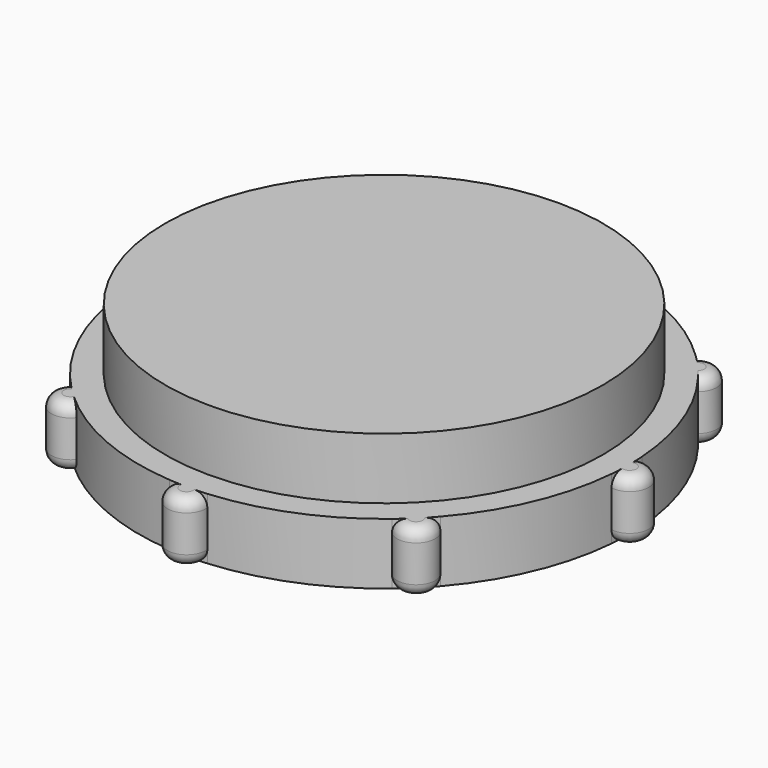
from build123d import *

# Parameters (mm, degrees)
F0_R         = 20
F1_DEPTH     = 5
F2_R         = 17.85
F3_DEPTH     = 5
F4_R         = 1.5514716271
F5_DEPTH     = 5
F6_T4_ANGLE  = 359.64
F6_S5_R      = 20
F6_T6_DEPTH  = 4
F6_T10_ANGLE = 359.64
F6_S11_R     = 20
F6_T12_DEPTH = 4
F6_T16_ANGLE = 359.64
F6_S17_R     = 20
F6_T18_DEPTH = 4
F6_T22_ANGLE = 359.64
F6_S23_R     = 20
F6_T24_DEPTH = 4
F6_T28_ANGLE = 359.64
F6_S29_R     = 20
F6_T30_DEPTH = 4
F6_T34_ANGLE = 359.64
F6_S35_R     = 20
F6_T36_DEPTH = 4
F6_T40_ANGLE = 359.64
F6_S41_R     = 20
F6_T42_DEPTH = 4
F6_T46_ANGLE = 359.64
F6_S47_R     = 20
F6_T48_DEPTH = 4
F6_T52_ANGLE = 359.64
F6_S53_R     = 20
F6_T54_DEPTH = 4
F6_T58_ANGLE = 359.64
F6_S59_R     = 20
F6_T60_DEPTH = 4
F6_T64_ANGLE = 359.64
F6_S65_R     = 20
F6_T66_DEPTH = 4
F6_T70_ANGLE = 359.64
F6_S71_R     = 20
F6_T72_DEPTH = 4
F6_T76_ANGLE = 359.64
F6_S77_R     = 20
F6_T78_DEPTH = 4
F6_T82_ANGLE = 359.64
F6_S83_R     = 20
F6_T84_DEPTH = 4
F6_T88_ANGLE = 359.64
F6_S89_R     = 20
F6_T90_DEPTH = 4
F6_T94_ANGLE = 359.64
F6_S95_R     = 20
F6_T96_DEPTH = 4


# Not quite as in the source:
# - a fillet or chamfer that OpenCascade refuses, or shapes differently, is made with other operations: its cross-section is extruded or revolved along the edge and cut away or added


with BuildPart() as f1:
    # F0 (on Top) → F1 (new body)
    with BuildSketch(Plane.XY):
        Circle(F0_R)
    extrude(amount=F1_DEPTH)

    # F2 (on face) → F3 (join)
    with BuildSketch(Plane.XY.offset(5)):
        Circle(F2_R)
    extrude(amount=F3_DEPTH)

    # F4 (on face) + F2 (on face) → F5 (join)
    with BuildSketch(Plane.XY):
        with Locations((0, -20.1228894293)):
            Circle(F4_R)
        with Locations((13.9962770045, -14.2214773223)):
            Circle(F4_R)
        with Locations((20.1879236847, -0.1935280598)):
            Circle(F4_R)
        with Locations((14.9637199938, 13.2539533079)):
            Circle(F4_R)
        with Locations((0.0650717993, 19.9293233454)):
            Circle(F4_R)
        with Locations((-13.8661321253, 14.6083775908)):
            Circle(F4_R)
        with Locations((-20.2512666583, -0.1935280598)):
            Circle(F4_R)
        with Locations((-13.962876983, -14.5117100328)):
            Circle(F4_R)
    with BuildSketch(Plane.XY.offset(5)):
        Circle(F2_R)
    extrude(amount=F5_DEPTH)

    # F6: fillet of radius 1 on 16 edges, made by hand


with BuildPart() as f6_tool2:
    # F6_s3 → F6_t4 (revolve)
    with BuildSketch(Plane(origin=(-0.0457273893, 0.0437221588, 0), x_dir=(0, 0, 1), z_dir=(0.7227767201, -0.6910816253, 0))):
        with BuildLine():
            ThreePointArc((0, 19.5867422733), (0.2928932188, 18.8796354921), (1, 18.5867422733))
            Line((1, 18.5867422733), (0, 18.5867422733))
            Line((0, 18.5867422733), (0, 19.5867422733))
        make_face()
    revolve(axis=Axis((-13.962876983, -14.5117100328, 0), (0, 0, 1)), revolution_arc=F6_T4_ANGLE)

    # F6_s5 → F6_t6 (cut, symmetric)
    with BuildSketch(Plane.XY.offset(0.5)):
        Circle(F6_S5_R)
    extrude(amount=F6_T6_DEPTH, both=True, mode=Mode.SUBTRACT)


with BuildPart() as f1_1:
    add(f1.part)

    # F6_t1: cut F6_tool2
    add(f6_tool2.part, mode=Mode.SUBTRACT)


with BuildPart() as f6_tool8:
    # F6_s9 → F6_t10 (revolve)
    with BuildSketch(Plane(origin=(0.0632175056, -0.0001986043, 0), x_dir=(0, 0, 1), z_dir=(-0.9999950652, 0.0031415875, 0))):
        with BuildLine():
            ThreePointArc((0, -19.5713184999), (0.2928932188, -18.8642117187), (1, -18.5713184999))
            Line((1, -18.5713184999), (0, -18.5713184999))
            Line((0, -18.5713184999), (0, -19.5713184999))
        make_face()
    revolve(axis=Axis((0, -20.1228894293, 0), (0, 0, -1)), revolution_arc=F6_T10_ANGLE)

    # F6_s11 → F6_t12 (cut, symmetric)
    with BuildSketch(Plane.XY.offset(0.5)):
        Circle(F6_S11_R)
    extrude(amount=F6_T12_DEPTH, both=True, mode=Mode.SUBTRACT)


with BuildPart() as f1_2:
    add(f1_1.part)

    # F6_t7: cut F6_tool8
    add(f6_tool8.part, mode=Mode.SUBTRACT)


with BuildPart() as f6_tool14:
    # F6_s15 → F6_t16 (revolve)
    with BuildSketch(Plane(origin=(0.044815932, 0.0438299518, 0), x_dir=(0, 0, 1), z_dir=(-0.7149274846, -0.6991986068, 0))):
        with BuildLine():
            ThreePointArc((0, -19.4020307643), (0.2928932188, -18.6949239831), (1, -18.4020307643))
            Line((1, -18.4020307643), (0, -18.4020307643))
            Line((0, -18.4020307643), (0, -19.4020307643))
        make_face()
    revolve(axis=Axis((13.9962770045, -14.2214773223, 0), (0, 0, -1)), revolution_arc=F6_T16_ANGLE)

    # F6_s17 → F6_t18 (cut, symmetric)
    with BuildSketch(Plane.XY.offset(0.5)):
        Circle(F6_S17_R)
    extrude(amount=F6_T18_DEPTH, both=True, mode=Mode.SUBTRACT)


with BuildPart() as f1_3:
    add(f1_2.part)

    # F6_t13: cut F6_tool14
    add(f6_tool14.part, mode=Mode.SUBTRACT)


with BuildPart() as f6_tool20:
    # F6_s21 → F6_t22 (revolve)
    with BuildSketch(Plane(origin=(0.0008072285, 0.0634199054, 0), x_dir=(0, 0, 1), z_dir=(-0.0127272835, -0.9999190048, 0))):
        with BuildLine():
            ThreePointArc((0, -19.6372800202), (0.2928932188, -18.930173239), (1, -18.6372800202))
            Line((1, -18.6372800202), (0, -18.6372800202))
            Line((0, -18.6372800202), (0, -19.6372800202))
        make_face()
    revolve(axis=Axis((20.1879236847, -0.1935280598, 0), (0, 0, -1)), revolution_arc=F6_T22_ANGLE)

    # F6_s23 → F6_t24 (cut, symmetric)
    with BuildSketch(Plane.XY.offset(0.5)):
        Circle(F6_S23_R)
    extrude(amount=F6_T24_DEPTH, both=True, mode=Mode.SUBTRACT)


with BuildPart() as f1_4:
    add(f1_3.part)

    # F6_t19: cut F6_tool20
    add(f6_tool20.part, mode=Mode.SUBTRACT)


with BuildPart() as f6_tool26:
    # F6_s27 → F6_t28 (revolve)
    with BuildSketch(Plane(origin=(-0.0414905629, 0.0471404143, 0), x_dir=(0, 0, 1), z_dir=(0.6606906965, -0.7506582469, 0))):
        with BuildLine():
            ThreePointArc((0, -19.4379318322), (0.2928932188, -18.730825051), (1, -18.4379318322))
            Line((1, -18.4379318322), (0, -18.4379318322))
            Line((0, -18.4379318322), (0, -19.4379318322))
        make_face()
    revolve(axis=Axis((14.9637199938, 13.2539533079, 0), (0, 0, -1)), revolution_arc=F6_T28_ANGLE)

    # F6_s29 → F6_t30 (cut, symmetric)
    with BuildSketch(Plane.XY.offset(0.5)):
        Circle(F6_S29_R)
    extrude(amount=F6_T30_DEPTH, both=True, mode=Mode.SUBTRACT)


with BuildPart() as f1_5:
    add(f1_4.part)

    # F6_t25: cut F6_tool26
    add(f6_tool26.part, mode=Mode.SUBTRACT)


with BuildPart() as f6_tool32:
    # F6_s33 → F6_t34 (revolve)
    with BuildSketch(Plane(origin=(0.0626100461, -7.7339e-06, 0), x_dir=(0, 0, 1), z_dir=(-0.9999999924, 0.0001235241, 0))):
        with BuildLine():
            ThreePointArc((0, 19.3778596043), (0.2928932188, 18.6707528231), (1, 18.3778596043))
            Line((1, 18.3778596043), (0, 18.3778596043))
            Line((0, 18.3778596043), (0, 19.3778596043))
        make_face()
    revolve(axis=Axis((0.0650717993, 19.9293233454, 0), (0, 0, 1)), revolution_arc=F6_T34_ANGLE)

    # F6_s35 → F6_t36 (cut, symmetric)
    with BuildSketch(Plane.XY.offset(0.5)):
        Circle(F6_S35_R)
    extrude(amount=F6_T36_DEPTH, both=True, mode=Mode.SUBTRACT)


with BuildPart() as f1_6:
    add(f1_5.part)

    # F6_t31: cut F6_tool32
    add(f6_tool32.part, mode=Mode.SUBTRACT)


with BuildPart() as f6_tool38:
    # F6_s39 → F6_t40 (revolve)
    with BuildSketch(Plane(origin=(0.045756417, 0.0437056306, 0), x_dir=(0, 0, 1), z_dir=(-0.7231261956, -0.6907159367, 0))):
        with BuildLine():
            ThreePointArc((0, 19.5897873236), (0.2928932188, 18.8826805424), (1, 18.5897873236))
            Line((1, 18.5897873236), (0, 18.5897873236))
            Line((0, 18.5897873236), (0, 19.5897873236))
        make_face()
    revolve(axis=Axis((-13.8661321253, 14.6083775908, 0), (0, 0, 1)), revolution_arc=F6_T40_ANGLE)

    # F6_s41 → F6_t42 (cut, symmetric)
    with BuildSketch(Plane.XY.offset(0.5)):
        Circle(F6_S41_R)
    extrude(amount=F6_T42_DEPTH, both=True, mode=Mode.SUBTRACT)


with BuildPart() as f1_7:
    add(f1_6.part)

    # F6_t37: cut F6_tool38
    add(f6_tool38.part, mode=Mode.SUBTRACT)


with BuildPart() as f6_tool44:
    # F6_s45 → F6_t46 (revolve)
    with BuildSketch(Plane(origin=(-0.0008078537, 0.0636189019, 0), x_dir=(0, 0, 1), z_dir=(0.012697304, -0.999919386, 0))):
        with BuildLine():
            ThreePointArc((0, 19.70061978), (0.2928932188, 18.9935129988), (1, 18.70061978))
            Line((1, 18.70061978), (0, 18.70061978))
            Line((0, 18.70061978), (0, 19.70061978))
        make_face()
    revolve(axis=Axis((-20.2512666583, -0.1935280598, 0), (0, 0, 1)), revolution_arc=F6_T46_ANGLE)

    # F6_s47 → F6_t48 (cut, symmetric)
    with BuildSketch(Plane.XY.offset(0.5)):
        Circle(F6_S47_R)
    extrude(amount=F6_T48_DEPTH, both=True, mode=Mode.SUBTRACT)


with BuildPart() as f1_8:
    add(f1_7.part)

    # F6_t43: cut F6_tool44
    add(f6_tool44.part, mode=Mode.SUBTRACT)


with BuildPart() as f6_tool50:
    # F6_s51 → F6_t52 (revolve)
    with BuildSketch(Plane(origin=(-0.0008078537, 0.0636189019, 0), x_dir=(0, 0, 1), z_dir=(0.012697304, -0.999919386, 0))):
        with BuildLine():
            ThreePointArc((5, 19.70061978), (4.7071067812, 18.9935129988), (4, 18.70061978))
            Line((4, 18.70061978), (5, 18.70061978))
            Line((5, 18.70061978), (5, 19.70061978))
        make_face()
    revolve(axis=Axis((-20.2512666583, -0.1935280598, 5), (0, 0, 1)), revolution_arc=F6_T52_ANGLE)

    # F6_s53 → F6_t54 (cut, symmetric)
    with BuildSketch(Plane.XY.offset(4.5)):
        Circle(F6_S53_R)
    extrude(amount=F6_T54_DEPTH, both=True, mode=Mode.SUBTRACT)


with BuildPart() as f1_9:
    add(f1_8.part)

    # F6_t49: cut F6_tool50
    add(f6_tool50.part, mode=Mode.SUBTRACT)


with BuildPart() as f6_tool56:
    # F6_s57 → F6_t58 (revolve)
    with BuildSketch(Plane(origin=(-0.0457273893, 0.0437221588, 0), x_dir=(0, 0, 1), z_dir=(0.7227767201, -0.6910816253, 0))):
        with BuildLine():
            ThreePointArc((5, 19.5867422733), (4.7071067812, 18.8796354921), (4, 18.5867422733))
            Line((4, 18.5867422733), (5, 18.5867422733))
            Line((5, 18.5867422733), (5, 19.5867422733))
        make_face()
    revolve(axis=Axis((-13.962876983, -14.5117100328, 5), (0, 0, 1)), revolution_arc=F6_T58_ANGLE)

    # F6_s59 → F6_t60 (cut, symmetric)
    with BuildSketch(Plane.XY.offset(4.5)):
        Circle(F6_S59_R)
    extrude(amount=F6_T60_DEPTH, both=True, mode=Mode.SUBTRACT)


with BuildPart() as f1_10:
    add(f1_9.part)

    # F6_t55: cut F6_tool56
    add(f6_tool56.part, mode=Mode.SUBTRACT)


with BuildPart() as f6_tool62:
    # F6_s63 → F6_t64 (revolve)
    with BuildSketch(Plane(origin=(-0.0632175056, -0.0001986043, 0), x_dir=(0, 0, 1), z_dir=(0.9999950652, 0.0031415875, 0))):
        with BuildLine():
            ThreePointArc((5, 19.5713184999), (4.7071067812, 18.8642117187), (4, 18.5713184999))
            Line((4, 18.5713184999), (5, 18.5713184999))
            Line((5, 18.5713184999), (5, 19.5713184999))
        make_face()
    revolve(axis=Axis((0, -20.1228894293, 5), (0, 0, 1)), revolution_arc=F6_T64_ANGLE)

    # F6_s65 → F6_t66 (cut, symmetric)
    with BuildSketch(Plane.XY.offset(4.5)):
        Circle(F6_S65_R)
    extrude(amount=F6_T66_DEPTH, both=True, mode=Mode.SUBTRACT)


with BuildPart() as f1_11:
    add(f1_10.part)

    # F6_t61: cut F6_tool62
    add(f6_tool62.part, mode=Mode.SUBTRACT)


with BuildPart() as f6_tool68:
    # F6_s69 → F6_t70 (revolve)
    with BuildSketch(Plane(origin=(-0.0445396574, -0.0441106716, 0), x_dir=(0, 0, 1), z_dir=(0.7105202071, 0.7036767975, 0))):
        with BuildLine():
            ThreePointArc((5, 19.4020307643), (4.7071067812, 18.6949239831), (4, 18.4020307643))
            Line((4, 18.4020307643), (5, 18.4020307643))
            Line((5, 18.4020307643), (5, 19.4020307643))
        make_face()
    revolve(axis=Axis((13.9962770045, -14.2214773223, 5), (0, 0, 1)), revolution_arc=F6_T70_ANGLE)

    # F6_s71 → F6_t72 (cut, symmetric)
    with BuildSketch(Plane.XY.offset(4.5)):
        Circle(F6_S71_R)
    extrude(amount=F6_T72_DEPTH, both=True, mode=Mode.SUBTRACT)


with BuildPart() as f1_12:
    add(f1_11.part)

    # F6_t67: cut F6_tool68
    add(f6_tool68.part, mode=Mode.SUBTRACT)


with BuildPart() as f6_tool74:
    # F6_s75 → F6_t76 (revolve)
    with BuildSketch(Plane(origin=(0.0008072285, 0.0634199054, 0), x_dir=(0, 0, 1), z_dir=(-0.0127272835, -0.9999190048, 0))):
        with BuildLine():
            ThreePointArc((5, -19.6372800202), (4.7071067812, -18.930173239), (4, -18.6372800202))
            Line((4, -18.6372800202), (5, -18.6372800202))
            Line((5, -18.6372800202), (5, -19.6372800202))
        make_face()
    revolve(axis=Axis((20.1879236847, -0.1935280598, 5), (0, 0, -1)), revolution_arc=F6_T76_ANGLE)

    # F6_s77 → F6_t78 (cut, symmetric)
    with BuildSketch(Plane.XY.offset(4.5)):
        Circle(F6_S77_R)
    extrude(amount=F6_T78_DEPTH, both=True, mode=Mode.SUBTRACT)


with BuildPart() as f1_13:
    add(f1_12.part)

    # F6_t73: cut F6_tool74
    add(f6_tool74.part, mode=Mode.SUBTRACT)


with BuildPart() as f6_tool80:
    # F6_s81 → F6_t82 (revolve)
    with BuildSketch(Plane(origin=(0.0417859339, -0.0468787926, 0), x_dir=(0, 0, 1), z_dir=(-0.6653941488, 0.7464922148, 0))):
        with BuildLine():
            ThreePointArc((5, 19.4379318322), (4.7071067812, 18.730825051), (4, 18.4379318322))
            Line((4, 18.4379318322), (5, 18.4379318322))
            Line((5, 18.4379318322), (5, 19.4379318322))
        make_face()
    revolve(axis=Axis((14.9637199938, 13.2539533079, 5), (0, 0, 1)), revolution_arc=F6_T82_ANGLE)

    # F6_s83 → F6_t84 (cut, symmetric)
    with BuildSketch(Plane.XY.offset(4.5)):
        Circle(F6_S83_R)
    extrude(amount=F6_T84_DEPTH, both=True, mode=Mode.SUBTRACT)


with BuildPart() as f1_14:
    add(f1_13.part)

    # F6_t79: cut F6_tool80
    add(f6_tool80.part, mode=Mode.SUBTRACT)


with BuildPart() as f6_tool86:
    # F6_s87 → F6_t88 (revolve)
    with BuildSketch(Plane(origin=(0.0626100461, -7.7339e-06, 0), x_dir=(0, 0, 1), z_dir=(-0.9999999924, 0.0001235241, 0))):
        with BuildLine():
            ThreePointArc((5, 19.3778596043), (4.7071067812, 18.6707528231), (4, 18.3778596043))
            Line((4, 18.3778596043), (5, 18.3778596043))
            Line((5, 18.3778596043), (5, 19.3778596043))
        make_face()
    revolve(axis=Axis((0.0650717993, 19.9293233454, 5), (0, 0, 1)), revolution_arc=F6_T88_ANGLE)

    # F6_s89 → F6_t90 (cut, symmetric)
    with BuildSketch(Plane.XY.offset(4.5)):
        Circle(F6_S89_R)
    extrude(amount=F6_T90_DEPTH, both=True, mode=Mode.SUBTRACT)


with BuildPart() as f1_15:
    add(f1_14.part)

    # F6_t85: cut F6_tool86
    add(f6_tool86.part, mode=Mode.SUBTRACT)


with BuildPart() as f6_tool92:
    # F6_s93 → F6_t94 (revolve)
    with BuildSketch(Plane(origin=(0.045756417, 0.0437056306, 0), x_dir=(0, 0, 1), z_dir=(-0.7231261956, -0.6907159367, 0))):
        with BuildLine():
            ThreePointArc((5, 19.5897873236), (4.7071067812, 18.8826805424), (4, 18.5897873236))
            Line((4, 18.5897873236), (5, 18.5897873236))
            Line((5, 18.5897873236), (5, 19.5897873236))
        make_face()
    revolve(axis=Axis((-13.8661321253, 14.6083775908, 5), (0, 0, 1)), revolution_arc=F6_T94_ANGLE)

    # F6_s95 → F6_t96 (cut, symmetric)
    with BuildSketch(Plane.XY.offset(4.5)):
        Circle(F6_S95_R)
    extrude(amount=F6_T96_DEPTH, both=True, mode=Mode.SUBTRACT)


with BuildPart() as f1_16:
    add(f1_15.part)

    # F6_t91: cut F6_tool92
    add(f6_tool92.part, mode=Mode.SUBTRACT)


solid = f1_16.part
